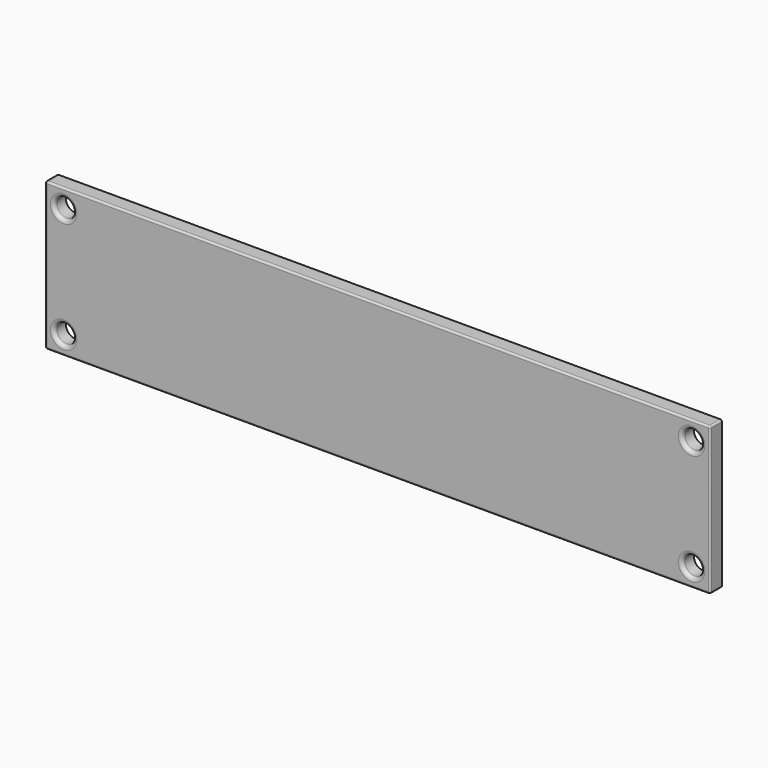
from build123d import *

# Parameters (mm, degrees)
F0_W         = 180
F0_H         = 40
F0_R         = 2.5751263091
F1_DEPTH     = 4
F2_R         = 1
F3_R         = 0.5
F4_TEXT_SIZE = 9.7585768742
F5_DEPTH     = 1


# Not quite as in the source:
# - a feature names something its author has since deleted; it is built from what else it names
# - Text() gives the source's letters only with a copy of the font that has no kerning and outlines rounded to 1/6400 em; it was checked with that copy


with BuildPart() as f1:
    # F0 (on Front) → F1 (new body)
    with BuildSketch(Plane.XZ):
        Rectangle(F0_W, F0_H)
        with Locations((-85, -15)):
            Circle(F0_R, mode=Mode.SUBTRACT)
        with Locations((85, -15)):
            Circle(F0_R, mode=Mode.SUBTRACT)
        with Locations((-85, 15)):
            Circle(F0_R, mode=Mode.SUBTRACT)
        with Locations((85, 15)):
            Circle(F0_R, mode=Mode.SUBTRACT)
    extrude(amount=F1_DEPTH)

    # F2
    f2_edges = [f1.edges().sort_by_distance(p)[0] for p in [
        (-87.575126, -4, 15),
        (-87.575126, -4, -15),
        (82.424874, -4, 15),
        (82.424874, -4, -15),
    ]]
    fillet(f2_edges, radius=F2_R)

    # F3
    f3_edges = [f1.edges().sort_by_distance(p)[0] for p in [
        (0, -4, 20),
        (-90, -4, 0),
        (0, -4, -20),
        (90, -4, 0),
        (-90, -2, 20),
        (-90, -2, -20),
        (90, -2, 20),
        (90, -2, -20),
    ]]
    fillet(f3_edges, radius=F3_R)

    # F4 (on face) → F5 (join)
    with BuildSketch(Plane(origin=(0, 0, 0), x_dir=(-1, 0, 0), z_dir=(0, 1, 0))):
        with Locations((-64.9919360876, -0.2709015603)):
            Text('Havana Body', F4_TEXT_SIZE, font='Open Sans', text_align=(TextAlign.LEFT, TextAlign.BOTTOM))
    extrude(amount=F5_DEPTH)

    # F6: F1 across plane


with BuildPart() as f1_1:
    add(f1.part)
    add(f1.part.mirror(Plane.YZ))


solid = f1_1.part
